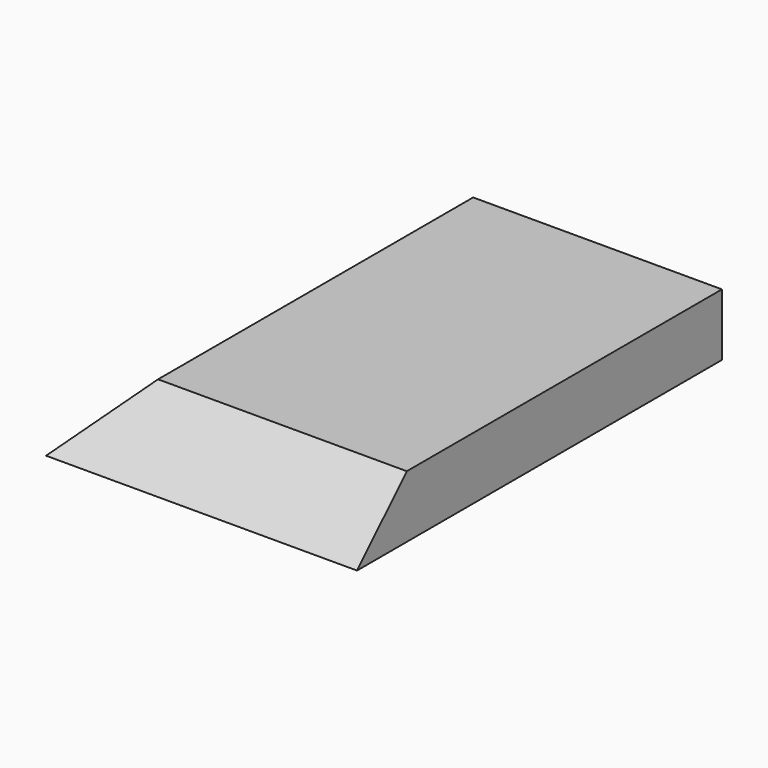
from build123d import *

# Parameters (mm, degrees)
F0_W     = 150
F0_H     = 220
F1_DEPTH = 30
F2_SIZE  = 29.99999


# Not quite as in the source:
# - a fillet or chamfer is up to 0.001 mm smaller than in the source, because OpenCascade refuses the exact size


with BuildPart() as f1:
    # F0 (on Top) → F1 (new body)
    with BuildSketch(Plane.XY):
        with Locations((4.4253946793, 0)):
            Rectangle(F0_W, F0_H)
    extrude(amount=F1_DEPTH)

    # F2 (size 30 in the source; OpenCascade refuses exactly that, so slightly less here)
    f2_edges = [f1.edges().sort_by_distance(p)[0] for p in [
        (4.425395, -110, 30),
        (-70.574605, 0, 30),
    ]]
    chamfer(f2_edges, length=F2_SIZE)


solid = f1.part
